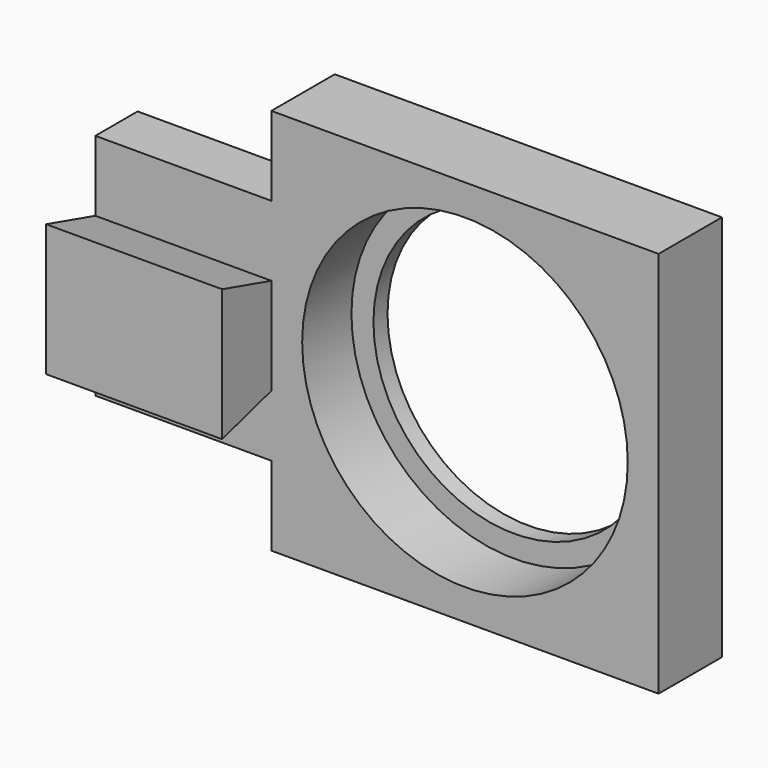
from build123d import *

# Parameters (mm, degrees)
F0_W      = 22
F0_H      = 22
F0_R      = 8
F1_DEPTH  = 1
F2_W      = 22
F2_H      = 22
F2_R      = 9.25
F3_DEPTH  = 3.5
F4_W      = 3
F4_H      = 13
F5_DEPTH  = 10
F6_W      = 10
F6_H      = 7.5
F7_DEPTH  = 3.5
F9_DEPTH  = 10
F10_DEPTH = 10


with BuildPart() as f1:
    # F0 (on Front) → F1 (new body)
    with BuildSketch(Plane.XZ):
        with Locations((11, 11)):
            Rectangle(F0_W, F0_H)
        with Locations((11, 11)):
            Circle(F0_R, mode=Mode.SUBTRACT)
    extrude(amount=F1_DEPTH)

    # F2 (on face) → F3 (join)
    with BuildSketch(Plane.XZ.offset(1)):
        with Locations((11, 11)):
            Rectangle(F2_W, F2_H)
        with Locations((11, 11)):
            Circle(F2_R, mode=Mode.SUBTRACT)
    extrude(amount=F3_DEPTH)

    # F4 (on face) → F5 (join)
    with BuildSketch(Plane(origin=(0, 0, 0), x_dir=(0, -1, 0), z_dir=(-1, 0, 0))):
        with Locations((3, 11)):
            Rectangle(F4_W, F4_H)
    extrude(amount=F5_DEPTH)

    # F6 (on face) → F7 (join)
    with BuildSketch(Plane.XZ.offset(4.5)):
        with Locations((-5, 10.75)):
            Rectangle(F6_W, F6_H)
    extrude(amount=F7_DEPTH)

    # F8 (on face) → F9 (cut)
    with BuildSketch(Plane(origin=(-10, 0, 0), x_dir=(0, -1, 0), z_dir=(-1, 0, 0))):
        Polygon((4.5, 7), (8, 7), (4.5, 8), align=None)
    extrude(amount=-F9_DEPTH, mode=Mode.SUBTRACT)

    # F8 (on face) → F10 (cut)
    with BuildSketch(Plane(origin=(-10, 0, 0), x_dir=(0, -1, 0), z_dir=(-1, 0, 0))):
        Polygon((4.5, 13.5), (8, 14.5), (4.5, 14.5), align=None)
    extrude(amount=-F10_DEPTH, mode=Mode.SUBTRACT)


solid = f1.part
